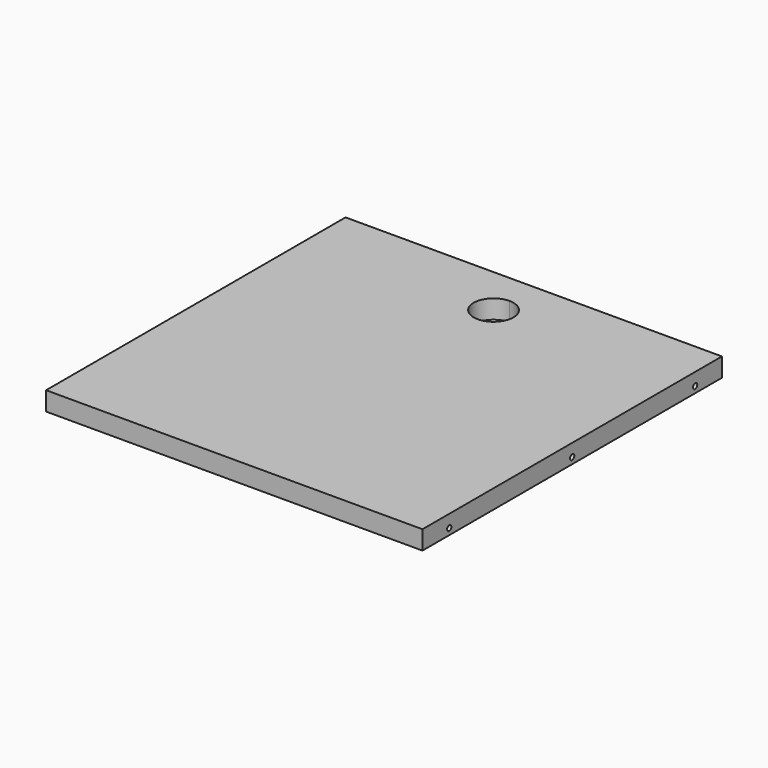
from build123d import *

# Parameters (mm, degrees)
F1_DEPTH  = 28.575
F3_D      = 15.0114
F3_DEPTH  = 14.224
F3_TIP    = 4.5098795482
F5_D      = 8.001
F5_DEPTH  = 25.4
F5_TIP    = 2.4037429064
F7_D      = 8.001
F7_DEPTH  = 25.4
F7_TIP    = 2.4037429064
F9_D      = 8.9916
F9_DEPTH  = 25.4
F9_TIP    = 2.701349171
F11_D     = 15.0114
F11_DEPTH = 14.224
F11_TIP   = 4.5098795482
F13_D     = 8.001
F13_DEPTH = 25.4
F13_TIP   = 2.4037429064


# Not quite as in the source:
# - a feature names something its author has since deleted; it is built from what else it names


with BuildPart() as f1:
    # F0 (on Top) → F1 (new body)
    with BuildSketch(Plane.XY):
        Polygon((285.75, -284.1625), (285.75, 284.1625), (0, 284.1625), (-285.75, 284.1625), (-285.75, -284.1625), align=None)
        with BuildLine():
            ThreePointArc((30.1625, 207.9625), (-21.3281082875, 186.6343917125), (0, 238.125))
            ThreePointArc((0, 238.125), (21.3281082875, 229.2906082875), (30.1625, 207.9625))
        make_face(mode=Mode.SUBTRACT)
    extrude(amount=F1_DEPTH)

    # F3
    with Locations(Plane(origin=(0, 0, 0), x_dir=(1, 0, 0), z_dir=(0, 0, -1))):
        with Locations((-261.874, 233.3625), (261.874, 233.3625), (-261.874, 0), (261.874, 0), (261.874, -233.3625), (-261.874, -233.3625)):
            Hole(F3_D / 2, depth=F3_DEPTH)
            with Locations((0, 0, -(F3_DEPTH + F3_TIP / 2))):  # 118° drill point
                Cone(0, F3_D / 2, F3_TIP, mode=Mode.SUBTRACT)

    # F5
    with Locations(Plane.YZ.offset(285.75)):
        with Locations((-233.3625, 9.525), (0, 9.525), (233.3625, 9.525)):
            Hole(F5_D / 2, depth=F5_DEPTH)
            with Locations((0, 0, -(F5_DEPTH + F5_TIP / 2))):  # 118° drill point
                Cone(0, F5_D / 2, F5_TIP, mode=Mode.SUBTRACT)

    # F7
    with Locations(Plane(origin=(-285.75, 0, 0), x_dir=(0, -1, 0), z_dir=(-1, 0, 0))):
        with Locations((0, 9.525), (233.3625, 9.525), (-233.3625, 9.525)):
            Hole(F7_D / 2, depth=F7_DEPTH)
            with Locations((0, 0, -(F7_DEPTH + F7_TIP / 2))):  # 118° drill point
                Cone(0, F7_D / 2, F7_TIP, mode=Mode.SUBTRACT)

    # F9
    with Locations(Plane(origin=(0, 0, 0), x_dir=(1, 0, 0), z_dir=(0, 0, -1))):
        with Locations((-228.6, -233.3625), (-184.15, -233.3625), (-184.15, -160.2105), (-228.6, -160.2105), (-228.6, 160.2105), (-228.6, 233.3625), (-184.15, 233.3625), (-184.15, 160.2105), (184.15, 233.3625), (228.6, 233.3625), (228.6, 160.2105), (184.15, 160.2105), (184.15, -160.2105), (228.6, -160.2105), (228.6, -233.3625), (184.15, -233.3625)):
            Hole(F9_D / 2, depth=F9_DEPTH)
            with Locations((0, 0, -(F9_DEPTH + F9_TIP / 2))):  # 118° drill point
                Cone(0, F9_D / 2, F9_TIP, mode=Mode.SUBTRACT)

    # F11
    with Locations(Plane(origin=(0, 0, 0), x_dir=(1, 0, 0), z_dir=(0, 0, -1))):
        with Locations((-234.95, -260.2865), (234.95, -260.2865)):
            Hole(F11_D / 2, depth=F11_DEPTH)
            with Locations((0, 0, -(F11_DEPTH + F11_TIP / 2))):  # 118° drill point
                Cone(0, F11_D / 2, F11_TIP, mode=Mode.SUBTRACT)

    # F13
    with Locations(Plane(origin=(0, 284.1625, 0), x_dir=(-1, 0, 0), z_dir=(0, 1, 0))):
        with Locations((-234.95, 9.525), (234.95, 9.525)):
            Hole(F13_D / 2, depth=F13_DEPTH)
            with Locations((0, 0, -(F13_DEPTH + F13_TIP / 2))):  # 118° drill point
                Cone(0, F13_D / 2, F13_TIP, mode=Mode.SUBTRACT)


solid = f1.part
